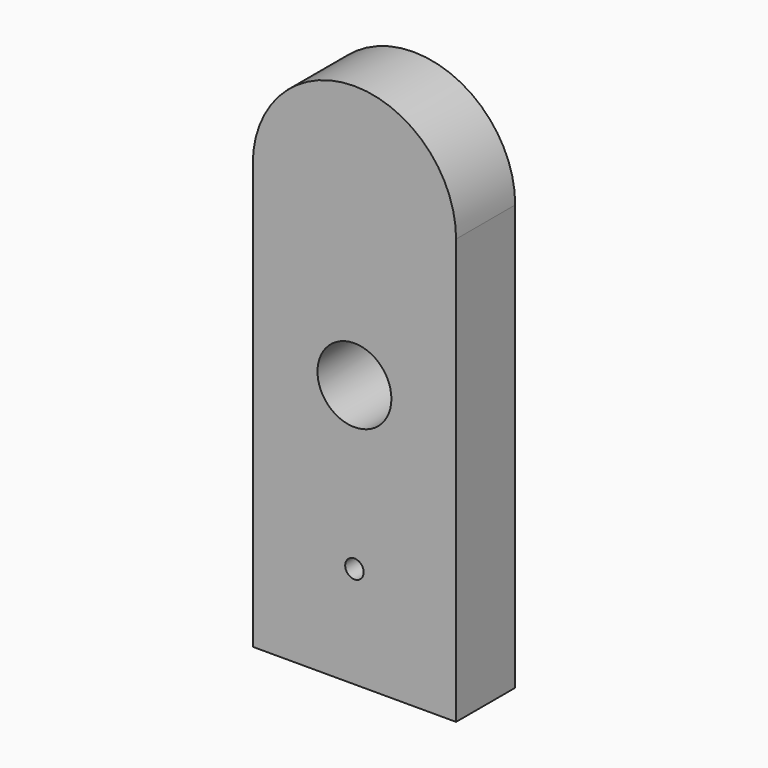
from build123d import *

# Parameters (mm, degrees)
F0_R     = 1
F0_R_2   = 4
F1_DEPTH = 8


# Not quite as in the source:
# - a feature names something its author has since deleted; it is built from what else it names


with BuildPart() as f1:
    # F0 (on Front) → F1 (new body)
    with BuildSketch(Plane.XZ):
        with BuildLine():
            Line((11, -17.5), (11, 17.5))
            ThreePointArc((11, 17.5), (0, 28.5), (-11, 17.5))
            Line((-11, 17.5), (-11, -17.5))
            Line((-11, -17.5), (-11, -28.5))
            Line((-11, -28.5), (0, -28.5))
            Line((0, -28.5), (11, -28.5))
            Line((11, -28.5), (11, -17.5))
        make_face()
        with Locations((0, -17.5)):
            Circle(F0_R, mode=Mode.SUBTRACT)
        Circle(F0_R_2, mode=Mode.SUBTRACT)
    extrude(amount=-F1_DEPTH)


solid = f1.part
